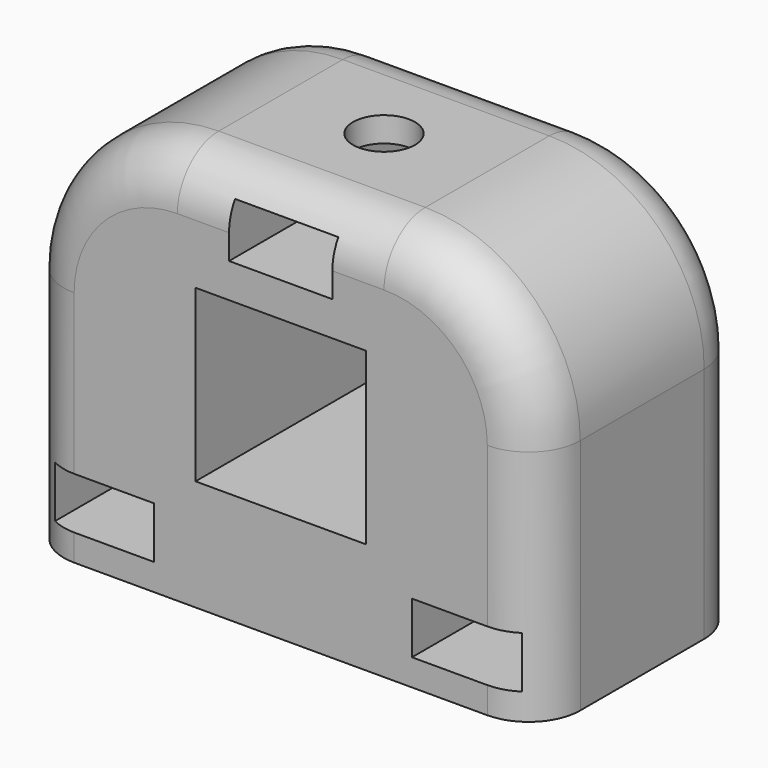
from build123d import *

# Parameters (mm, degrees)
F0_W         = 50
F0_H         = 38
F0_W_2       = 10
F0_H_2       = 5
F0_W_3       = 16.5
F0_H_3       = 16.5
F1_DEPTH     = 25
F2_R         = 3
F3_DEPTH     = 7.4141664952
F4_R         = 3
F5_DEPTH     = 7.571767807
F6_R         = 15
F7_T1_DEPTH  = 35.5
F7_T3_DEPTH  = 20
F7_T6_ANGLE  = 90
F7_T8_ANGLE  = 90
F7_T10_ANGLE = 90
F7_T12_ANGLE = 90


# Not quite as in the source:
# - a fillet or chamfer that OpenCascade refuses, or shapes differently, is made with other operations: its cross-section is extruded or revolved along the edge and cut away or added


with BuildPart() as f1:
    # F0 (on Front) → F1 (new body)
    with BuildSketch(Plane.XZ):
        Rectangle(F0_W, F0_H)
        with Locations((-17.2914686799, -13.928232193)):
            Rectangle(F0_W_2, F0_H_2, mode=Mode.SUBTRACT)
        with Locations((17.7085313201, -13.928232193)):
            Rectangle(F0_W_2, F0_H_2, mode=Mode.SUBTRACT)
        Rectangle(F0_W_3, F0_H_3, mode=Mode.SUBTRACT)
        with Locations((0, 14.0858335048)):
            Rectangle(F0_W_2, F0_H_2, mode=Mode.SUBTRACT)
    extrude(amount=F1_DEPTH)

    # F2 (on face) → F3 (cut, through all)
    with BuildSketch(Plane.XY.offset(19)):
        with Locations((0, -12.5)):
            Circle(F2_R)
    extrude(amount=-F3_DEPTH, mode=Mode.SUBTRACT)

    # F4 (on face) → F5 (cut, through all)
    with BuildSketch(Plane(origin=(0, 0, -19), x_dir=(1, 0, 0), z_dir=(0, 0, -1))):
        with Locations((-17.2914686799, 11)):
            Circle(F4_R)
        with Locations((17.7085313201, 11)):
            Circle(F4_R)
    extrude(amount=-F5_DEPTH, mode=Mode.SUBTRACT)

    # F6
    f6_edges = [f1.edges().sort_by_distance(p)[0] for p in [
        (-25, -12.5, 19),
        (25, -12.5, 19),
    ]]
    fillet(f6_edges, radius=F6_R)

    # F7: fillet of radius 5 on 10 edges, made by hand

    # F7_s2 → F7_t1 (cut)
    with BuildSketch(Plane.XY.offset(-31.5)):
        with BuildLine():
            ThreePointArc((-20, 0), (-23.5355339059, -1.4644660941), (-25, -5))
            Line((-25, -5), (-25, 0))
            Line((-25, 0), (-20, 0))
        make_face()
        with BuildLine():
            ThreePointArc((20, 0), (23.5355339059, -1.4644660941), (25, -5))
            Line((25, -5), (25, 0))
            Line((25, 0), (20, 0))
        make_face()
        with BuildLine():
            ThreePointArc((20, -25), (23.5355339059, -23.5355339059), (25, -20))
            Line((25, -20), (25, -25))
            Line((25, -25), (20, -25))
        make_face()
        with BuildLine():
            ThreePointArc((-20, -25), (-23.5355339059, -23.5355339059), (-25, -20))
            Line((-25, -20), (-25, -25))
            Line((-25, -25), (-20, -25))
        make_face()
    extrude(amount=F7_T1_DEPTH, mode=Mode.SUBTRACT)

    # F7_s4 → F7_t3 (cut)
    with BuildSketch(Plane.YZ.offset(-10)):
        with BuildLine():
            ThreePointArc((-20, 19), (-23.5355339059, 17.5355339059), (-25, 14))
            Line((-25, 14), (-25, 19))
            Line((-25, 19), (-20, 19))
        make_face()
        with BuildLine():
            ThreePointArc((-5, 19), (-1.4644660941, 17.5355339059), (0, 14))
            Line((0, 14), (0, 19))
            Line((0, 19), (-5, 19))
        make_face()
    extrude(amount=F7_T3_DEPTH, mode=Mode.SUBTRACT)

    # F7_s5 → F7_t6 (revolve, cut)
    with BuildSketch(Plane.YZ.offset(-10)):
        with BuildLine():
            ThreePointArc((0, 14), (-1.4644660941, 17.5355339059), (-5, 19))
            Line((-5, 19), (0, 19))
            Line((0, 19), (0, 14))
        make_face()
    revolve(axis=Axis((-10, 0, 4), (0, -1, 0)), revolution_arc=F7_T6_ANGLE, mode=Mode.SUBTRACT)

    # F7_s7 → F7_t8 (revolve, cut)
    with BuildSketch(Plane.YZ.offset(10)):
        with BuildLine():
            ThreePointArc((0, 14), (-1.4644660941, 17.5355339059), (-5, 19))
            Line((-5, 19), (0, 19))
            Line((0, 19), (0, 14))
        make_face()
    revolve(axis=Axis((10, 0, 4), (0, 1, 0)), revolution_arc=F7_T8_ANGLE, mode=Mode.SUBTRACT)

    # F7_s9 → F7_t10 (revolve, cut)
    with BuildSketch(Plane.YZ.offset(10)):
        with BuildLine():
            ThreePointArc((-20, 19), (-23.5355339059, 17.5355339059), (-25, 14))
            Line((-25, 14), (-25, 19))
            Line((-25, 19), (-20, 19))
        make_face()
    revolve(axis=Axis((10, -25, 4), (0, 1, 0)), revolution_arc=F7_T10_ANGLE, mode=Mode.SUBTRACT)

    # F7_s11 → F7_t12 (revolve, cut)
    with BuildSketch(Plane.YZ.offset(-10)):
        with BuildLine():
            ThreePointArc((-20, 19), (-23.5355339059, 17.5355339059), (-25, 14))
            Line((-25, 14), (-25, 19))
            Line((-25, 19), (-20, 19))
        make_face()
    revolve(axis=Axis((-10, -25, 4), (0, -1, 0)), revolution_arc=F7_T12_ANGLE, mode=Mode.SUBTRACT)


solid = f1.part
